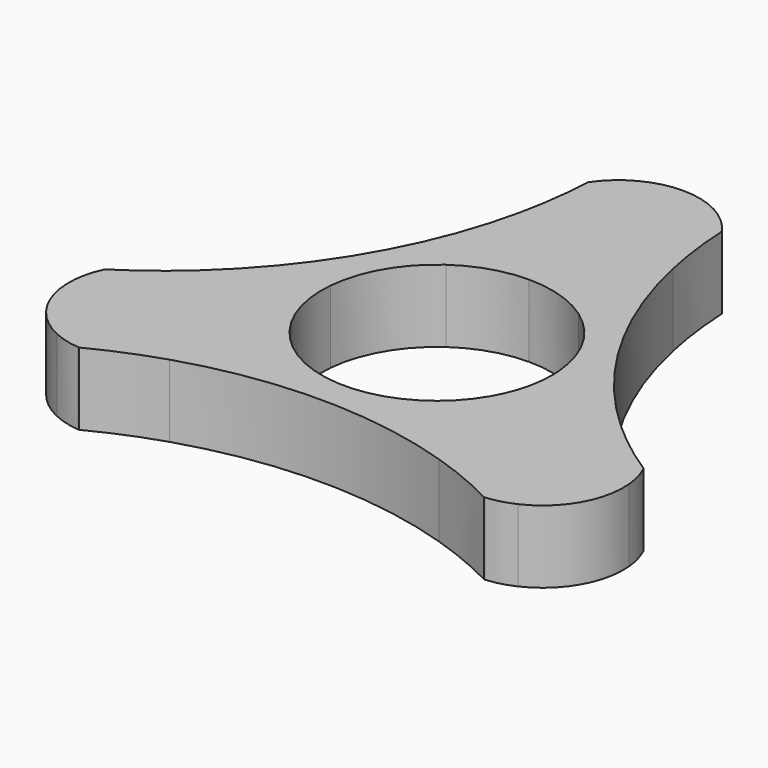
from build123d import *

# Parameters (mm, degrees)
F1_DEPTH = 6.9342


with BuildPart() as f1:
    # F0 (on Top) → F1 (new body)
    with BuildSketch(Plane.XY):
        with BuildLine():
            ThreePointArc((10.978713393, 0.9937852859), (11.0123726308, 0.4973992365), (11.0236, 0))
            ThreePointArc((11.0236, 0), (10.6479799387, -2.8531176256), (9.5467176412, -5.5118))
            ThreePointArc((9.5467176412, -5.5118), (7.4352089911, -8.1386377373), (4.628713393, -10.0047373422))
            Line((4.628713393, -10.0047373422), (11.7777531012, -14.1322373422))
            ThreePointArc((11.7777531012, -14.1322373422), (12.0895321135, -6.9798946201), (18.1277531012, -3.1337147141))
            Line((18.1277531012, -3.1337147141), (10.978713393, 0.9937852859))
        make_face()
        with BuildLine():
            ThreePointArc((6.35, 9.0109520562), (9.5467176412, 5.5118), (10.978713393, 0.9937852859))
            Line((10.978713393, 0.9937852859), (18.1277531012, -3.1337147141))
            ThreePointArc((18.1277531012, -3.1337147141), (19.1741700395, -3.1132418489), (20.2138057566, -3.2339278992))
            ThreePointArc((20.2138057566, -3.2339278992), (12.0108278998, 6.9344547212), (7.3062391636, 19.1226332419))
            ThreePointArc((7.3062391636, 19.1226332419), (6.8909384905, 18.1619392751), (6.35, 17.2659520562))
            Line((6.35, 17.2659520562), (6.35, 9.0109520562))
        make_face()
        with BuildLine():
            ThreePointArc((0, 11.0236), (3.3306625371, 10.5083987374), (6.35, 9.0109520562))
            Line((6.35, 9.0109520562), (6.35, 17.2659520562))
            ThreePointArc((6.35, 17.2659520562), (0, 13.9597892403), (-6.35, 17.2659520562))
            Line((-6.35, 17.2659520562), (-6.35, 9.0109520562))
            ThreePointArc((-6.35, 9.0109520562), (-3.3306625371, 10.5083987374), (0, 11.0236))
        make_face()
        with BuildLine():
            ThreePointArc((20.2138057566, -3.2339278992), (19.1741700395, -3.1132418489), (18.1277531012, -3.1337147141))
            Line((18.1277531012, -3.1337147141), (25.8267189409, -7.5787147141))
            ThreePointArc((25.8267189409, -7.5787147141), (25.8095339268, -7.5421240909), (25.7921583133, -7.5056235914))
            ThreePointArc((25.7921583133, -7.5056235914), (22.9140380361, -5.4859265713), (20.2138057566, -3.2339278992))
        make_face()
        with BuildLine():
            Line((25.8267189409, -7.5787147141), (18.1277531012, -3.1337147141))
            ThreePointArc((18.1277531012, -3.1337147141), (12.0895321135, -6.9798946201), (11.7777531012, -14.1322373422))
            Line((11.7777531012, -14.1322373422), (19.4767189409, -18.5772373422))
            ThreePointArc((19.4767189409, -18.5772373422), (20.8083845795, -18.3425243759), (22.0789973351, -17.8799589479))
            Line((22.0789973351, -17.8799589479), (26.5239973351, -10.1809931083))
            ThreePointArc((26.5239973351, -10.1809931083), (26.2892843688, -8.8493274697), (25.8267189409, -7.5787147141))
        make_face()
        with BuildLine():
            Line((11.7777531012, -14.1322373422), (4.628713393, -10.0047373422))
            ThreePointArc((4.628713393, -10.0047373422), (0, -11.0236), (-4.628713393, -10.0047373422))
            Line((-4.628713393, -10.0047373422), (-11.7777531012, -14.1322373422))
            ThreePointArc((-11.7777531012, -14.1322373422), (-12.283231549, -15.0486974262), (-12.907566593, -15.8887053427))
            ThreePointArc((-12.907566593, -15.8887053427), (0, -13.8689094423), (12.907566593, -15.8887053427))
            ThreePointArc((12.907566593, -15.8887053427), (12.283231549, -15.0486974262), (11.7777531012, -14.1322373422))
        make_face()
        with BuildLine():
            ThreePointArc((-6.35, 17.2659520562), (0, 13.9597892403), (6.35, 17.2659520562))
            Line((6.35, 17.2659520562), (6.35, 26.1559520562))
            ThreePointArc((6.35, 26.1559520562), (5.4808997893, 27.1918518455), (4.445, 28.0609520562))
            Line((4.445, 28.0609520562), (-4.445, 28.0609520562))
            ThreePointArc((-4.445, 28.0609520562), (-5.4808997893, 27.1918518455), (-6.35, 26.1559520562))
            Line((-6.35, 26.1559520562), (-6.35, 17.2659520562))
        make_face()
        with BuildLine():
            Line((6.35, 26.1559520562), (6.35, 17.2659520562))
            ThreePointArc((6.35, 17.2659520562), (6.8909384905, 18.1619392751), (7.3062391636, 19.1226332419))
            ThreePointArc((7.3062391636, 19.1226332419), (6.706067244, 22.5871023282), (6.3960184553, 26.0894761135))
            ThreePointArc((6.3960184553, 26.0894761135), (6.3730959022, 26.1227740859), (6.35, 26.1559520562))
        make_face()
        with BuildLine():
            Line((19.4767189409, -18.5772373422), (11.7777531012, -14.1322373422))
            ThreePointArc((11.7777531012, -14.1322373422), (12.283231549, -15.0486974262), (12.907566593, -15.8887053427))
            ThreePointArc((12.907566593, -15.8887053427), (16.2079707921, -17.1011757569), (19.3961398581, -18.5838525221))
            ThreePointArc((19.3961398581, -18.5838525221), (19.4364380247, -18.580649995), (19.4767189409, -18.5772373422))
        make_face()
        with BuildLine():
            Line((-11.7777531012, -14.1322373422), (-4.628713393, -10.0047373422))
            ThreePointArc((-4.628713393, -10.0047373422), (-7.4352089911, -8.1386377373), (-9.5467176412, -5.5118))
            ThreePointArc((-9.5467176412, -5.5118), (-10.7658715282, -2.3697610001), (-10.978713393, 0.9937852859))
            Line((-10.978713393, 0.9937852859), (-18.1277531012, -3.1337147141))
            ThreePointArc((-18.1277531012, -3.1337147141), (-12.0895321135, -6.9798946201), (-11.7777531012, -14.1322373422))
        make_face()
        with BuildLine():
            ThreePointArc((-10.978713393, 0.9937852859), (-9.5467176412, 5.5118), (-6.35, 9.0109520562))
            Line((-6.35, 9.0109520562), (-6.35, 17.2659520562))
            ThreePointArc((-6.35, 17.2659520562), (-6.8909384905, 18.1619392751), (-7.3062391636, 19.1226332419))
            ThreePointArc((-7.3062391636, 19.1226332419), (-12.0108278998, 6.9344547212), (-20.2138057566, -3.2339278992))
            ThreePointArc((-20.2138057566, -3.2339278992), (-19.1741700395, -3.1132418489), (-18.1277531012, -3.1337147141))
            Line((-18.1277531012, -3.1337147141), (-10.978713393, 0.9937852859))
        make_face()
        with BuildLine():
            ThreePointArc((-7.3062391636, 19.1226332419), (-6.8909384905, 18.1619392751), (-6.35, 17.2659520562))
            Line((-6.35, 17.2659520562), (-6.35, 26.1559520562))
            ThreePointArc((-6.35, 26.1559520562), (-6.3730959022, 26.1227740859), (-6.3960184553, 26.0894761135))
            ThreePointArc((-6.3960184553, 26.0894761135), (-6.706067244, 22.5871023282), (-7.3062391636, 19.1226332419))
        make_face()
        with BuildLine():
            ThreePointArc((22.0789973351, -17.8799589479), (25.5149399286, -14.7310574361), (26.5239973351, -10.1809931083))
            Line((26.5239973351, -10.1809931083), (22.0789973351, -17.8799589479))
        make_face()
        with BuildLine():
            ThreePointArc((-12.907566593, -15.8887053427), (-12.283231549, -15.0486974262), (-11.7777531012, -14.1322373422))
            Line((-11.7777531012, -14.1322373422), (-19.4767189409, -18.5772373422))
            ThreePointArc((-19.4767189409, -18.5772373422), (-19.4364380247, -18.580649995), (-19.3961398581, -18.5838525221))
            ThreePointArc((-19.3961398581, -18.5838525221), (-16.2079707921, -17.1011757569), (-12.907566593, -15.8887053427))
        make_face()
        with BuildLine():
            Line((-19.4767189409, -18.5772373422), (-11.7777531012, -14.1322373422))
            ThreePointArc((-11.7777531012, -14.1322373422), (-12.0895321135, -6.9798946201), (-18.1277531012, -3.1337147141))
            Line((-18.1277531012, -3.1337147141), (-25.8267189409, -7.5787147141))
            ThreePointArc((-25.8267189409, -7.5787147141), (-26.2892843688, -8.8493274697), (-26.5239973351, -10.1809931083))
            Line((-26.5239973351, -10.1809931083), (-22.0789973351, -17.8799589479))
            ThreePointArc((-22.0789973351, -17.8799589479), (-20.8083845795, -18.3425243759), (-19.4767189409, -18.5772373422))
        make_face()
        with BuildLine():
            Line((-4.445, 28.0609520562), (4.445, 28.0609520562))
            ThreePointArc((4.445, 28.0609520562), (0, 29.4621148722), (-4.445, 28.0609520562))
        make_face()
        with BuildLine():
            Line((-25.8267189409, -7.5787147141), (-18.1277531012, -3.1337147141))
            ThreePointArc((-18.1277531012, -3.1337147141), (-19.1741700395, -3.1132418489), (-20.2138057566, -3.2339278992))
            ThreePointArc((-20.2138057566, -3.2339278992), (-22.9140380361, -5.4859265713), (-25.7921583133, -7.5056235914))
            ThreePointArc((-25.7921583133, -7.5056235914), (-25.8095339268, -7.5421240909), (-25.8267189409, -7.5787147141))
        make_face()
        with BuildLine():
            ThreePointArc((-26.5239973351, -10.1809931083), (-25.5149399286, -14.7310574361), (-22.0789973351, -17.8799589479))
            Line((-22.0789973351, -17.8799589479), (-26.5239973351, -10.1809931083))
        make_face()
    extrude(amount=F1_DEPTH)


solid = f1.part
